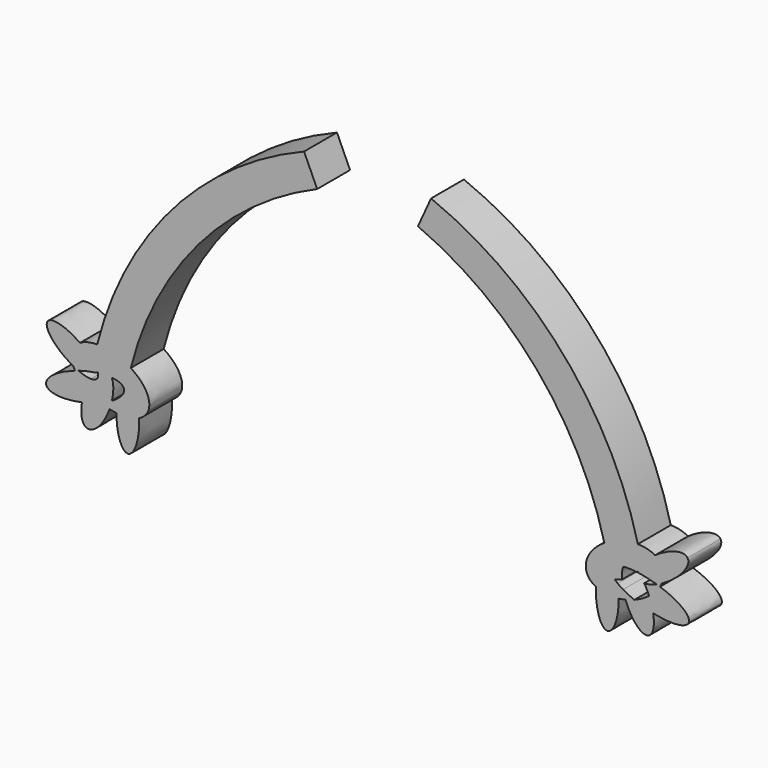
from build123d import *

# Parameters (mm, degrees)
F1_DEPTH = 5.588


with BuildPart() as f1:
    # F0 (on Front) → F1 (new body)
    with BuildSketch(Plane.XZ):
        with BuildLine():
            Line((32.2706997395, 11.8237007409), (36.8935018778, 12.8905009478))
            ThreePointArc((36.8935018778, 12.8905009478), (36.8110087462, 13.2342292177), (36.7259397745, 13.5773290723))
            add(Edge.make_bspline(
                [(36.7259397745, 13.5773290723), (34.3340010738, 13.6080468465), (32.1682575581, 12.2374034623)],
                knots=[4.1398736957, 4.1398736957, 4.1398736957, 5.0351295074, 5.0351295074, 5.0351295074], degree=2, weights=[1, 0.9014763473, 1]))
            ThreePointArc((32.1682575581, 12.2374034623), (32.2199801898, 12.0306762946), (32.2706997395, 11.8237007409))
        make_face()
        with BuildLine():
            ThreePointArc((36.7259397745, 13.5773290723), (36.8110087462, 13.2342292177), (36.8935018778, 12.8905009478))
            Line((36.8935018778, 12.8905009478), (32.2706997395, 11.8237007409))
            ThreePointArc((32.2706997395, 11.8237007409), (32.2199801898, 12.0306762946), (32.1682575581, 12.2374034623))
            add(Edge.make_bspline(
                [(32.1682575581, 12.2374034623), (28.9205076549, 10.1819860565), (29.7814980149, 7.9121002927)],
                knots=[5.0351295074, 5.0351295074, 5.0351295074, 6.2831853072, 6.2831853072, 6.2831853072], degree=2, weights=[1, 0.8115315094, 1]))
            add(Edge.make_bspline(
                [(29.7814980149, 7.9121002927), (30.0935316875, 7.0894653085), (31.0231862525, 6.6210745378)],
                knots=[0, 0, 0, 0.5104960555, 0.5104960555, 0.5104960555], degree=2, weights=[1, 0.9676007021, 1]))
            add(Edge.make_bspline(
                [(31.0231862525, 6.6210745378), (32.2803370197, 5.9876803301), (34.1259638549, 6.2135645276)],
                knots=[0.5104960555, 0.5104960555, 0.5104960555, 1.1889418798, 1.1889418798, 1.1889418798], degree=2, weights=[1, 0.9430135296, 1]))
            add(Edge.make_bspline(
                [(34.1259638549, 6.2135645276), (34.1243304614, 7.1393539704), (33.986892498, 7.9823561587)],
                knots=[1.5757090143, 1.5757090143, 1.5757090143, 1.9969423736, 1.9969423736, 1.9969423736], degree=2, weights=[1, 0.9779021758, 1]))
            add(Edge.make_bspline(
                [(33.5814264788, 8.3342957348), (33.7569586016, 8.1594602494), (33.986892498, 7.9823561587)],
                knots=[3.6789423363, 3.6789423363, 3.6789423363, 3.8326748164, 3.8326748164, 3.8326748164], degree=2, weights=[1, 0.9970472448, 1]))
            ThreePointArc((33.5814264788, 8.3342957349), (33.7430587819, 8.3767272254), (33.9042244499, 8.4208980334))
            ThreePointArc((33.9042244499, 8.4208980334), (34.2272864678, 8.5151058653), (34.5482281316, 8.6163018704))
            add(Edge.make_bspline(
                [(34.7502826908, 10.2419972443), (34.4767828785, 9.6352454307), (34.5482281316, 8.6163018704)],
                knots=[3.5532795904, 3.5532795904, 3.5532795904, 4.1157635759, 4.1157635759, 4.1157635759], degree=2, weights=[1, 0.9607114655, 1]))
            add(Edge.make_bspline(
                [(36.6366435764, 10.182329208), (35.5729011314, 10.3132979273), (34.7502826908, 10.2419972443)],
                knots=[1.9968428936, 1.9968428936, 1.9968428936, 2.4151242253, 2.4151242253, 2.4151242253], degree=2, weights=[1, 0.9782096903, 1]))
            add(Edge.make_bspline(
                [(36.6736091343, 10.3151708305), (36.6517615378, 10.247208944), (36.6366435764, 10.182329208)],
                knots=[2.6853839142, 2.6853839142, 2.6853839142, 2.7479252243, 2.7479252243, 2.7479252243], degree=2, weights=[1, 0.9995111129, 1]))
            add(Edge.make_bspline(
                [(39.0587814304, 13.001263099), (37.0867427344, 11.6003162638), (36.6736091343, 10.3151708305)],
                knots=[1.6170702637, 1.6170702637, 1.6170702637, 2.6853839142, 2.6853839142, 2.6853839142], degree=2, weights=[1, 0.8606982085, 1]))
            add(Edge.make_bspline(
                [(39.0587814304, 13.001263099), (38.1255784861, 13.559354621), (36.7259397745, 13.5773290723)],
                knots=[3.5920969612, 3.5920969612, 3.5920969612, 4.1398736957, 4.1398736957, 4.1398736957], degree=2, weights=[1, 0.9627264634, 1]))
        make_face()
        with BuildLine():
            add(Edge.make_bspline(
                [(36.7259397745, 13.5773290723), (34.3340010738, 13.6080468465), (32.1682575581, 12.2374034623)],
                knots=[4.1398736957, 4.1398736957, 4.1398736957, 5.0351295074, 5.0351295074, 5.0351295074], degree=2, weights=[1, 0.9014763473, 1]))
            ThreePointArc((36.7259397745, 13.5773290723), (26.5357798175, 33.0496078391), (8.6232991889, 45.7835011184))
            Line((8.6232991889, 45.7835011184), (6.8453005515, 41.8718978763))
            ThreePointArc((6.8453005515, 41.8718978763), (22.9723649253, 30.0160267189), (32.1682575581, 12.2374034623))
        make_face()
        with BuildLine():
            add(Edge.make_bspline(
                [(43.4721000493, 14.1350999475), (42.5506163385, 15.4818812905), (39.0587814304, 13.001263099)],
                knots=[0, 0, 0, 1.6170702637, 1.6170702637, 1.6170702637], degree=2, weights=[1, 0.690558678, 1]))
            add(Edge.make_bspline(
                [(39.9796777774, 9.9352008957), (40.8468053822, 11.9319554905), (39.0587814304, 13.001263099)],
                knots=[2.604464445, 2.604464445, 2.604464445, 3.5920969612, 3.5920969612, 3.5920969612], degree=2, weights=[1, 0.8805304081, 1]))
            add(Edge.make_bspline(
                [(39.9796777774, 9.9352008957), (44.6497104326, 12.413980328), (43.4721000493, 14.1350999475)],
                knots=[4.4248856689, 4.4248856689, 4.4248856689, 6.2831853072, 6.2831853072, 6.2831853072], degree=2, weights=[1, 0.5985152881, 1]))
        make_face()
        with BuildLine():
            add(Edge.make_bspline(
                [(39.9796777774, 9.9352008957), (40.8468053822, 11.9319554905), (39.0587814304, 13.001263099)],
                knots=[2.604464445, 2.604464445, 2.604464445, 3.5920969612, 3.5920969612, 3.5920969612], degree=2, weights=[1, 0.8805304081, 1]))
            add(Edge.make_bspline(
                [(39.0587814304, 13.001263099), (37.0867427344, 11.6003162638), (36.6736091343, 10.3151708305)],
                knots=[1.6170702637, 1.6170702637, 1.6170702637, 2.6853839142, 2.6853839142, 2.6853839142], degree=2, weights=[1, 0.8606982085, 1]))
            add(Edge.make_bspline(
                [(36.838546125, 10.1558680731), (36.7561354159, 10.2402088688), (36.6736091343, 10.3151708305)],
                knots=[2.3750268658, 2.3750268658, 2.3750268658, 2.4506633861, 2.4506633861, 2.4506633861], degree=2, weights=[1, 0.9992849748, 1]))
            add(Edge.make_bspline(
                [(37.6420765384, 10.020492761), (37.2334774045, 10.1010140748), (36.838546125, 10.1558680731)],
                knots=[1.8015665825, 1.8015665825, 1.8015665825, 1.9568242788, 1.9568242788, 1.9568242788], degree=2, weights=[1, 0.9969883938, 1]))
            add(Edge.make_bspline(
                [(39.2873464103, 9.604313109), (38.467052792, 9.8579173509), (37.6420765384, 10.020492761)],
                knots=[1.4900094279, 1.4900094279, 1.4900094279, 1.8015665825, 1.8015665825, 1.8015665825], degree=2, weights=[1, 0.9878910345, 1]))
            add(Edge.make_bspline(
                [(39.2873464103, 9.604313109), (39.6288573586, 9.748990969), (39.9796777774, 9.9352008957)],
                knots=[4.2244590735, 4.2244590735, 4.2244590735, 4.4248856689, 4.4248856689, 4.4248856689], degree=2, weights=[1, 0.9949828484, 1]))
        make_face()
        with BuildLine():
            add(Edge.make_bspline(
                [(39.7319677558, 9.459773657), (39.8761405135, 9.6967832669), (39.9796777774, 9.9352008957)],
                knots=[2.4760921827, 2.4760921827, 2.4760921827, 2.604464445, 2.604464445, 2.604464445], degree=2, weights=[1, 0.9979407774, 1]))
            add(Edge.make_bspline(
                [(39.2873464103, 9.604313109), (39.6288573586, 9.748990969), (39.9796777774, 9.9352008957)],
                knots=[4.2244590735, 4.2244590735, 4.2244590735, 4.4248856689, 4.4248856689, 4.4248856689], degree=2, weights=[1, 0.9949828484, 1]))
            add(Edge.make_bspline(
                [(39.7319677558, 9.459773657), (39.5117613547, 9.5349323646), (39.2873464103, 9.604313109)],
                knots=[1.4041305877, 1.4041305877, 1.4041305877, 1.4900094279, 1.4900094279, 1.4900094279], degree=2, weights=[1, 0.9990782447, 1]))
        make_face()
        with BuildLine():
            add(Edge.make_bspline(
                [(38.8016372647, 5.9750217773), (43.2541867053, 5.0072999504), (43.6518237169, 6.4967344439), (44.0494607285, 7.9861689374), (39.7319677558, 9.459773657)],
                knots=[4.8870250081, 4.8870250081, 4.8870250081, 6.2871704515, 6.2871704515, 7.6873158949, 7.6873158949, 7.6873158949], degree=2, weights=[1, 0.7647953367, 1, 0.7647953367, 1]))
            add(Edge.make_bspline(
                [(38.2513832681, 7.8754265107), (39.210650648, 8.6027659512), (39.7319677558, 9.459773657)],
                knots=[2.019377813, 2.019377813, 2.019377813, 2.4760921827, 2.4760921827, 2.4760921827], degree=2, weights=[1, 0.9740396059, 1]))
            add(Edge.make_bspline(
                [(38.8016372647, 5.9750217773), (38.6410074231, 6.9230354431), (38.2513832681, 7.8754265107)],
                knots=[1.1577399392, 1.1577399392, 1.1577399392, 1.650437424, 1.650437424, 1.650437424], degree=2, weights=[1, 0.9698092967, 1]))
        make_face()
        with BuildLine():
            add(Edge.make_bspline(
                [(38.2513832681, 7.8754265107), (39.210650648, 8.6027659512), (39.7319677558, 9.459773657)],
                knots=[2.019377813, 2.019377813, 2.019377813, 2.4760921827, 2.4760921827, 2.4760921827], degree=2, weights=[1, 0.9740396059, 1]))
            add(Edge.make_bspline(
                [(39.7319677558, 9.459773657), (39.5117613547, 9.5349323646), (39.2873464103, 9.604313109)],
                knots=[1.4041305877, 1.4041305877, 1.4041305877, 1.4900094279, 1.4900094279, 1.4900094279], degree=2, weights=[1, 0.9990782447, 1]))
            add(Edge.make_bspline(
                [(37.5898259242, 9.1787969257), (38.2981843104, 9.1852640083), (39.2873464103, 9.604313109)],
                knots=[3.6576642826, 3.6576642826, 3.6576642826, 4.2244590735, 4.2244590735, 4.2244590735], degree=2, weights=[1, 0.9601110043, 1]))
            add(Edge.make_bspline(
                [(38.2513832681, 7.8754265107), (37.9624894998, 8.5815938285), (37.5898259242, 9.1787969257)],
                knots=[1.650437424, 1.650437424, 1.650437424, 2.0190978507, 2.0190978507, 2.0190978507], degree=2, weights=[1, 0.9830592351, 1]))
        make_face()
        with BuildLine():
            add(Edge.make_bspline(
                [(31.0231862525, 6.6210745378), (32.2803370197, 5.9876803301), (34.1259638549, 6.2135645276)],
                knots=[0.5104960555, 0.5104960555, 0.5104960555, 1.1889418798, 1.1889418798, 1.1889418798], degree=2, weights=[1, 0.9430135296, 1]))
            add(Edge.make_bspline(
                [(31.0231862525, 6.6210745378), (30.8609649248, 2.0815590872), (32.4974887078, 1.866622695), (34.1340124909, 1.6516863028), (34.1259638549, 6.2135645276)],
                knots=[4.613210998, 4.613210998, 4.613210998, 6.2360526598, 6.2360526598, 7.8588943215, 7.8588943215, 7.8588943215], degree=2, weights=[1, 0.6884686478, 1, 0.6884686478, 1]))
        make_face()
        with BuildLine():
            add(Edge.make_bspline(
                [(38.8016372647, 5.9750217773), (38.6410074231, 6.9230354431), (38.2513832681, 7.8754265107)],
                knots=[1.1577399392, 1.1577399392, 1.1577399392, 1.650437424, 1.650437424, 1.650437424], degree=2, weights=[1, 0.9698092967, 1]))
            add(Edge.make_bspline(
                [(36.2437126455, 6.7579420356), (37.3562007183, 7.196677719), (38.2513832681, 7.8754265107)],
                knots=[1.5922240618, 1.5922240618, 1.5922240618, 2.019377813, 2.019377813, 2.019377813], degree=2, weights=[1, 0.9772790247, 1]))
            add(Edge.make_bspline(
                [(36.2437126455, 6.7579420356), (37.4688080387, 6.2647002976), (38.8016372647, 5.9750217773)],
                knots=[4.3929880742, 4.3929880742, 4.3929880742, 4.8870250081, 4.8870250081, 4.8870250081], degree=2, weights=[1, 0.9696457571, 1]))
        make_face()
        with BuildLine():
            add(Edge.make_bspline(
                [(35.0496863908, 6.3809924019), (36.1985024094, 3.2377777269), (37.7606059218, 3.068754155), (39.3227094342, 2.899730583), (38.8016372647, 5.9750217773)],
                knots=[4.703944968, 4.703944968, 4.703944968, 6.0724351072, 6.0724351072, 7.4409252464, 7.4409252464, 7.4409252464], degree=2, weights=[1, 0.7748964505, 1, 0.7748964505, 1]))
            add(Edge.make_bspline(
                [(36.2437126455, 6.7579420356), (37.4688080387, 6.2647002976), (38.8016372647, 5.9750217773)],
                knots=[4.3929880742, 4.3929880742, 4.3929880742, 4.8870250081, 4.8870250081, 4.8870250081], degree=2, weights=[1, 0.9696457571, 1]))
            add(Edge.make_bspline(
                [(35.0496863908, 6.3809924019), (35.6560069837, 6.5261665663), (36.2437126455, 6.7579420356)],
                knots=[1.3640671148, 1.3640671148, 1.3640671148, 1.5922240618, 1.5922240618, 1.5922240618], degree=2, weights=[1, 0.9935001046, 1]))
        make_face()
        with BuildLine():
            add(Edge.make_bspline(
                [(34.1259638549, 6.2135645276), (34.1243304614, 7.1393539704), (33.986892498, 7.9823561587)],
                knots=[1.5757090143, 1.5757090143, 1.5757090143, 1.9969423736, 1.9969423736, 1.9969423736], degree=2, weights=[1, 0.9779021758, 1]))
            add(Edge.make_bspline(
                [(34.1259638549, 6.2135645276), (34.58512877, 6.2697612063), (35.0496863908, 6.3809924019)],
                knots=[1.1889418798, 1.1889418798, 1.1889418798, 1.3640671148, 1.3640671148, 1.3640671148], degree=2, weights=[1, 0.9961688428, 1]))
            add(Edge.make_bspline(
                [(34.7193628832, 7.4945536546), (34.8463562994, 6.9373130979), (35.0496863908, 6.3809924019)],
                knots=[4.4171809306, 4.4171809306, 4.4171809306, 4.703944968, 4.703944968, 4.703944968], degree=2, weights=[1, 0.9897383966, 1]))
            add(Edge.make_bspline(
                [(33.986892498, 7.9823561587), (34.3069609657, 7.7358268919), (34.7193628832, 7.4945536546)],
                knots=[3.8326748164, 3.8326748164, 3.8326748164, 4.0462773342, 4.0462773342, 4.0462773342], degree=2, weights=[1, 0.9943021647, 1]))
        make_face()
        with BuildLine():
            add(Edge.make_bspline(
                [(35.0496863908, 6.3809924019), (35.6560069837, 6.5261665663), (36.2437126455, 6.7579420356)],
                knots=[1.3640671148, 1.3640671148, 1.3640671148, 1.5922240618, 1.5922240618, 1.5922240618], degree=2, weights=[1, 0.9935001046, 1]))
            add(Edge.make_bspline(
                [(34.7193628832, 7.4945536546), (35.3929708023, 7.1004634325), (36.2437126455, 6.7579420356)],
                knots=[4.0462773342, 4.0462773342, 4.0462773342, 4.3929880742, 4.3929880742, 4.3929880742], degree=2, weights=[1, 0.9850115505, 1]))
            add(Edge.make_bspline(
                [(34.7193628832, 7.4945536546), (34.8463562994, 6.9373130979), (35.0496863908, 6.3809924019)],
                knots=[4.4171809306, 4.4171809306, 4.4171809306, 4.703944968, 4.703944968, 4.703944968], degree=2, weights=[1, 0.9897383966, 1]))
        make_face()
    extrude(amount=F1_DEPTH)


with BuildPart() as f1b:
    # F0 (on Front) → F1, piece 2 (new body)
    with BuildSketch(Plane.XZ):
        with BuildLine():
            Line((-32.2706997395, 11.8237007409), (-36.8935018778, 12.8905009478))
            ThreePointArc((-36.8935018778, 12.8905009478), (-36.8110087462, 13.2342292177), (-36.7259397745, 13.5773290723))
            add(Edge.make_bspline(
                [(-36.7259397745, 13.5773290723), (-38.1255784861, 13.559354621), (-39.0587814304, 13.001263099)],
                knots=[2.1433116115, 2.1433116115, 2.1433116115, 2.691088346, 2.691088346, 2.691088346], degree=2, weights=[1, 0.9627264634, 1]))
            add(Edge.make_bspline(
                [(-36.6736091343, 10.3151708305), (-37.0867427344, 11.6003162638), (-39.0587814304, 13.001263099)],
                knots=[3.5978013929, 3.5978013929, 3.5978013929, 4.6661150434, 4.6661150434, 4.6661150434], degree=2, weights=[1, 0.8606982085, 1]))
            add(Edge.make_bspline(
                [(-36.6366435764, 10.182329208), (-36.6517615378, 10.247208944), (-36.6736091343, 10.3151708305)],
                knots=[3.5352600828, 3.5352600828, 3.5352600828, 3.5978013929, 3.5978013929, 3.5978013929], degree=2, weights=[1, 0.9995111129, 1]))
            add(Edge.make_bspline(
                [(-37.5898259242, 9.1787969257), (-36.4002747552, 9.167936709), (-36.6366435764, 10.182329208)],
                knots=[2.6255210246, 2.6255210246, 2.6255210246, 3.5352600828, 3.5352600828, 3.5352600828], degree=2, weights=[1, 0.8983183576, 1]))
            add(Edge.make_bspline(
                [(-37.5898259242, 9.1787969257), (-37.9624894998, 8.5815938285), (-38.2513832681, 7.8754265107)],
                knots=[4.2640874565, 4.2640874565, 4.2640874565, 4.6327478832, 4.6327478832, 4.6327478832], degree=2, weights=[1, 0.9830592351, 1]))
            add(Edge.make_bspline(
                [(-38.2513832681, 7.8754265107), (-37.3562007183, 7.196677719), (-36.2437126455, 6.7579420356)],
                knots=[4.2638074942, 4.2638074942, 4.2638074942, 4.6909612454, 4.6909612454, 4.6909612454], degree=2, weights=[1, 0.9772790247, 1]))
            add(Edge.make_bspline(
                [(-36.2437126455, 6.7579420356), (-35.3929708023, 7.1004634325), (-34.7193628832, 7.4945536546)],
                knots=[1.8901972329, 1.8901972329, 1.8901972329, 2.2369079729, 2.2369079729, 2.2369079729], degree=2, weights=[1, 0.9850115505, 1]))
            add(Edge.make_bspline(
                [(-34.7193628832, 7.4945536546), (-34.3138711823, 9.2738303121), (-34.7502826908, 10.2419972443)],
                knots=[1.8660043766, 1.8660043766, 1.8660043766, 2.7299057168, 2.7299057168, 2.7299057168], degree=2, weights=[1, 0.9081508434, 1]))
            add(Edge.make_bspline(
                [(-33.986892498, 7.9823561587), (-31.4271573207, 9.9539644252), (-34.7502826908, 10.2419972443)],
                knots=[2.4505104908, 2.4505104908, 2.4505104908, 3.8680610818, 3.8680610818, 3.8680610818], degree=2, weights=[1, 0.7591596108, 1]))
            add(Edge.make_bspline(
                [(-33.986892498, 7.9823561587), (-34.1243304614, 7.1393539704), (-34.1259638549, 6.2135645276)],
                knots=[4.2862429336, 4.2862429336, 4.2862429336, 4.7074762928, 4.7074762928, 4.7074762928], degree=2, weights=[1, 0.9779021758, 1]))
            add(Edge.make_bspline(
                [(-34.1259638549, 6.2135645276), (-32.2803370197, 5.9876803301), (-31.0231862525, 6.6210745378)],
                knots=[5.0942434274, 5.0942434274, 5.0942434274, 5.7726892517, 5.7726892517, 5.7726892517], degree=2, weights=[1, 0.9430135296, 1]))
            add(Edge.make_bspline(
                [(-31.0231862525, 6.6210745378), (-30.0935316875, 7.0894653085), (-29.7814980149, 7.9121002927)],
                knots=[5.7726892517, 5.7726892517, 5.7726892517, 6.2831853072, 6.2831853072, 6.2831853072], degree=2, weights=[1, 0.9676007021, 1]))
            add(Edge.make_bspline(
                [(-29.7814980149, 7.9121002927), (-28.9205076549, 10.1819860565), (-32.1682575581, 12.2374034623)],
                knots=[0, 0, 0, 1.2480557998, 1.2480557998, 1.2480557998], degree=2, weights=[1, 0.8115315094, 1]))
            ThreePointArc((-32.1682575581, 12.2374034623), (-32.2199801898, 12.0306762946), (-32.2706997395, 11.8237007409))
        make_face()
        with BuildLine():
            ThreePointArc((-36.7259397745, 13.5773290723), (-36.8110087462, 13.2342292177), (-36.8935018778, 12.8905009478))
            Line((-36.8935018778, 12.8905009478), (-32.2706997395, 11.8237007409))
            ThreePointArc((-32.2706997395, 11.8237007409), (-32.2199801898, 12.0306762946), (-32.1682575581, 12.2374034623))
            add(Edge.make_bspline(
                [(-32.1682575581, 12.2374034623), (-34.3340010738, 13.6080468465), (-36.7259397745, 13.5773290723)],
                knots=[1.2480557998, 1.2480557998, 1.2480557998, 2.1433116115, 2.1433116115, 2.1433116115], degree=2, weights=[1, 0.9014763473, 1]))
        make_face()
        with BuildLine():
            ThreePointArc((-8.6232991889, 45.7835011184), (-26.5357798175, 33.0496078391), (-36.7259397745, 13.5773290723))
            add(Edge.make_bspline(
                [(-32.1682575581, 12.2374034623), (-34.3340010738, 13.6080468465), (-36.7259397745, 13.5773290723)],
                knots=[1.2480557998, 1.2480557998, 1.2480557998, 2.1433116115, 2.1433116115, 2.1433116115], degree=2, weights=[1, 0.9014763473, 1]))
            ThreePointArc((-32.1682575581, 12.2374034623), (-22.9723649253, 30.0160267189), (-6.8453005515, 41.8718978763))
            Line((-6.8453005515, 41.8718978763), (-8.6232991889, 45.7835011184))
        make_face()
        with BuildLine():
            add(Edge.make_bspline(
                [(-36.6736091343, 10.3151708305), (-37.0867427344, 11.6003162638), (-39.0587814304, 13.001263099)],
                knots=[3.5978013929, 3.5978013929, 3.5978013929, 4.6661150434, 4.6661150434, 4.6661150434], degree=2, weights=[1, 0.8606982085, 1]))
            add(Edge.make_bspline(
                [(-39.0587814304, 13.001263099), (-39.8198979479, 12.5460859285), (-40.0939062238, 11.8236998096)],
                knots=[2.691088346, 2.691088346, 2.691088346, 3.1415926536, 3.1415926536, 3.1415926536], degree=2, weights=[1, 0.974737819, 1]))
            add(Edge.make_bspline(
                [(-40.0939062238, 11.8236998096), (-40.4230078995, 10.9560673212), (-39.9796777774, 9.9352008957)],
                knots=[3.1415926536, 3.1415926536, 3.1415926536, 3.6787208622, 3.6787208622, 3.6787208622], degree=2, weights=[1, 0.9641529012, 1]))
            add(Edge.make_bspline(
                [(-39.9796777774, 9.9352008957), (-39.6288573586, 9.748990969), (-39.2873464103, 9.604313109)],
                knots=[1.8582996383, 1.8582996383, 1.8582996383, 2.0587262337, 2.0587262337, 2.0587262337], degree=2, weights=[1, 0.9949828484, 1]))
            add(Edge.make_bspline(
                [(-36.838546125, 10.1558680731), (-38.045603473, 9.9882137871), (-39.2873464103, 9.604313109)],
                knots=[4.3263610283, 4.3263610283, 4.3263610283, 4.7931758793, 4.7931758793, 4.7931758793], degree=2, weights=[1, 0.9728839277, 1]))
            add(Edge.make_bspline(
                [(-36.6736091343, 10.3151708305), (-36.7561354159, 10.2402088688), (-36.838546125, 10.1558680731)],
                knots=[3.8325219211, 3.8325219211, 3.8325219211, 3.9081584414, 3.9081584414, 3.9081584414], degree=2, weights=[1, 0.9992849748, 1]))
        make_face()
        with BuildLine():
            add(Edge.make_bspline(
                [(-39.0587814304, 13.001263099), (-39.8198979479, 12.5460859285), (-40.0939062238, 11.8236998096)],
                knots=[2.691088346, 2.691088346, 2.691088346, 3.1415926536, 3.1415926536, 3.1415926536], degree=2, weights=[1, 0.974737819, 1]))
            add(Edge.make_bspline(
                [(-39.0587814304, 13.001263099), (-42.5506163385, 15.4818812905), (-43.4721000493, 14.1350999475)],
                knots=[4.6661150434, 4.6661150434, 4.6661150434, 6.2831853072, 6.2831853072, 6.2831853072], degree=2, weights=[1, 0.690558678, 1]))
            add(Edge.make_bspline(
                [(-43.4721000493, 14.1350999475), (-44.6497104326, 12.413980328), (-39.9796777774, 9.9352008957)],
                knots=[0, 0, 0, 1.8582996383, 1.8582996383, 1.8582996383], degree=2, weights=[1, 0.5985152881, 1]))
            add(Edge.make_bspline(
                [(-40.0939062238, 11.8236998096), (-40.4230078995, 10.9560673212), (-39.9796777774, 9.9352008957)],
                knots=[3.1415926536, 3.1415926536, 3.1415926536, 3.6787208622, 3.6787208622, 3.6787208622], degree=2, weights=[1, 0.9641529012, 1]))
        make_face()
        with BuildLine():
            add(Edge.make_bspline(
                [(-34.1259638549, 6.2135645276), (-34.1340124909, 1.6516863028), (-32.4974887078, 1.866622695), (-30.8609649248, 2.0815590872), (-31.0231862525, 6.6210745378)],
                knots=[4.7074762928, 4.7074762928, 4.7074762928, 6.3303179546, 6.3303179546, 7.9531596163, 7.9531596163, 7.9531596163], degree=2, weights=[1, 0.6884686478, 1, 0.6884686478, 1]))
            add(Edge.make_bspline(
                [(-34.1259638549, 6.2135645276), (-32.2803370197, 5.9876803301), (-31.0231862525, 6.6210745378)],
                knots=[5.0942434274, 5.0942434274, 5.0942434274, 5.7726892517, 5.7726892517, 5.7726892517], degree=2, weights=[1, 0.9430135296, 1]))
        make_face()
        with BuildLine():
            add(Edge.make_bspline(
                [(-39.9796777774, 9.9352008957), (-39.6288573586, 9.748990969), (-39.2873464103, 9.604313109)],
                knots=[1.8582996383, 1.8582996383, 1.8582996383, 2.0587262337, 2.0587262337, 2.0587262337], degree=2, weights=[1, 0.9949828484, 1]))
            add(Edge.make_bspline(
                [(-39.9796777774, 9.9352008957), (-39.8761405135, 9.6967832669), (-39.7319677558, 9.459773657)],
                knots=[3.6787208622, 3.6787208622, 3.6787208622, 3.8070931244, 3.8070931244, 3.8070931244], degree=2, weights=[1, 0.9979407774, 1]))
            add(Edge.make_bspline(
                [(-39.2873464103, 9.604313109), (-39.5117613547, 9.5349323646), (-39.7319677558, 9.459773657)],
                knots=[4.7931758793, 4.7931758793, 4.7931758793, 4.8790547195, 4.8790547195, 4.8790547195], degree=2, weights=[1, 0.9990782447, 1]))
        make_face()
        with BuildLine():
            add(Edge.make_bspline(
                [(-35.0496863908, 6.3809924019), (-34.58512877, 6.2697612063), (-34.1259638549, 6.2135645276)],
                knots=[4.9191181924, 4.9191181924, 4.9191181924, 5.0942434274, 5.0942434274, 5.0942434274], degree=2, weights=[1, 0.9961688428, 1]))
            add(Edge.make_bspline(
                [(-33.986892498, 7.9823561587), (-34.1243304614, 7.1393539704), (-34.1259638549, 6.2135645276)],
                knots=[4.2862429336, 4.2862429336, 4.2862429336, 4.7074762928, 4.7074762928, 4.7074762928], degree=2, weights=[1, 0.9779021758, 1]))
            add(Edge.make_bspline(
                [(-34.7193628832, 7.4945536546), (-34.3069609657, 7.7358268919), (-33.986892498, 7.9823561587)],
                knots=[2.2369079729, 2.2369079729, 2.2369079729, 2.4505104908, 2.4505104908, 2.4505104908], degree=2, weights=[1, 0.9943021647, 1]))
            add(Edge.make_bspline(
                [(-35.0496863908, 6.3809924019), (-34.8463562994, 6.9373130979), (-34.7193628832, 7.4945536546)],
                knots=[1.5792403392, 1.5792403392, 1.5792403392, 1.8660043766, 1.8660043766, 1.8660043766], degree=2, weights=[1, 0.9897383966, 1]))
        make_face()
        with BuildLine():
            add(Edge.make_bspline(
                [(-39.7319677558, 9.459773657), (-39.210650648, 8.6027659512), (-38.2513832681, 7.8754265107)],
                knots=[3.8070931244, 3.8070931244, 3.8070931244, 4.2638074942, 4.2638074942, 4.2638074942], degree=2, weights=[1, 0.9740396059, 1]))
            add(Edge.make_bspline(
                [(-39.7319677558, 9.459773657), (-44.0494607285, 7.9861689374), (-43.6518237169, 6.4967344439), (-43.2541867053, 5.0072999504), (-38.8016372647, 5.9750217773)],
                knots=[4.8790547195, 4.8790547195, 4.8790547195, 6.2792001629, 6.2792001629, 7.6793456062, 7.6793456062, 7.6793456062], degree=2, weights=[1, 0.7647953367, 1, 0.7647953367, 1]))
            add(Edge.make_bspline(
                [(-38.2513832681, 7.8754265107), (-38.6410074231, 6.9230354431), (-38.8016372647, 5.9750217773)],
                knots=[4.6327478832, 4.6327478832, 4.6327478832, 5.125445368, 5.125445368, 5.125445368], degree=2, weights=[1, 0.9698092967, 1]))
        make_face()
        with BuildLine():
            add(Edge.make_bspline(
                [(-39.2873464103, 9.604313109), (-39.5117613547, 9.5349323646), (-39.7319677558, 9.459773657)],
                knots=[4.7931758793, 4.7931758793, 4.7931758793, 4.8790547195, 4.8790547195, 4.8790547195], degree=2, weights=[1, 0.9990782447, 1]))
            add(Edge.make_bspline(
                [(-39.7319677558, 9.459773657), (-39.210650648, 8.6027659512), (-38.2513832681, 7.8754265107)],
                knots=[3.8070931244, 3.8070931244, 3.8070931244, 4.2638074942, 4.2638074942, 4.2638074942], degree=2, weights=[1, 0.9740396059, 1]))
            add(Edge.make_bspline(
                [(-37.5898259242, 9.1787969257), (-37.9624894998, 8.5815938285), (-38.2513832681, 7.8754265107)],
                knots=[4.2640874565, 4.2640874565, 4.2640874565, 4.6327478832, 4.6327478832, 4.6327478832], degree=2, weights=[1, 0.9830592351, 1]))
            add(Edge.make_bspline(
                [(-39.2873464103, 9.604313109), (-38.2981843104, 9.1852640083), (-37.5898259242, 9.1787969257)],
                knots=[2.0587262337, 2.0587262337, 2.0587262337, 2.6255210246, 2.6255210246, 2.6255210246], degree=2, weights=[1, 0.9601110043, 1]))
        make_face()
        with BuildLine():
            add(Edge.make_bspline(
                [(-38.8016372647, 5.9750217773), (-39.3227094342, 2.899730583), (-37.7606059218, 3.068754155), (-36.1985024094, 3.2377777269), (-35.0496863908, 6.3809924019)],
                knots=[5.125445368, 5.125445368, 5.125445368, 6.4939355072, 6.4939355072, 7.8624256464, 7.8624256464, 7.8624256464], degree=2, weights=[1, 0.7748964505, 1, 0.7748964505, 1]))
            add(Edge.make_bspline(
                [(-36.2437126455, 6.7579420356), (-35.6560069837, 6.5261665663), (-35.0496863908, 6.3809924019)],
                knots=[4.6909612454, 4.6909612454, 4.6909612454, 4.9191181924, 4.9191181924, 4.9191181924], degree=2, weights=[1, 0.9935001046, 1]))
            add(Edge.make_bspline(
                [(-38.8016372647, 5.9750217773), (-37.4688080387, 6.2647002976), (-36.2437126455, 6.7579420356)],
                knots=[1.3961602991, 1.3961602991, 1.3961602991, 1.8901972329, 1.8901972329, 1.8901972329], degree=2, weights=[1, 0.9696457571, 1]))
        make_face()
        with BuildLine():
            add(Edge.make_bspline(
                [(-36.2437126455, 6.7579420356), (-35.6560069837, 6.5261665663), (-35.0496863908, 6.3809924019)],
                knots=[4.6909612454, 4.6909612454, 4.6909612454, 4.9191181924, 4.9191181924, 4.9191181924], degree=2, weights=[1, 0.9935001046, 1]))
            add(Edge.make_bspline(
                [(-35.0496863908, 6.3809924019), (-34.8463562994, 6.9373130979), (-34.7193628832, 7.4945536546)],
                knots=[1.5792403392, 1.5792403392, 1.5792403392, 1.8660043766, 1.8660043766, 1.8660043766], degree=2, weights=[1, 0.9897383966, 1]))
            add(Edge.make_bspline(
                [(-36.2437126455, 6.7579420356), (-35.3929708023, 7.1004634325), (-34.7193628832, 7.4945536546)],
                knots=[1.8901972329, 1.8901972329, 1.8901972329, 2.2369079729, 2.2369079729, 2.2369079729], degree=2, weights=[1, 0.9850115505, 1]))
        make_face()
        with BuildLine():
            add(Edge.make_bspline(
                [(-38.2513832681, 7.8754265107), (-38.6410074231, 6.9230354431), (-38.8016372647, 5.9750217773)],
                knots=[4.6327478832, 4.6327478832, 4.6327478832, 5.125445368, 5.125445368, 5.125445368], degree=2, weights=[1, 0.9698092967, 1]))
            add(Edge.make_bspline(
                [(-38.8016372647, 5.9750217773), (-37.4688080387, 6.2647002976), (-36.2437126455, 6.7579420356)],
                knots=[1.3961602991, 1.3961602991, 1.3961602991, 1.8901972329, 1.8901972329, 1.8901972329], degree=2, weights=[1, 0.9696457571, 1]))
            add(Edge.make_bspline(
                [(-38.2513832681, 7.8754265107), (-37.3562007183, 7.196677719), (-36.2437126455, 6.7579420356)],
                knots=[4.2638074942, 4.2638074942, 4.2638074942, 4.6909612454, 4.6909612454, 4.6909612454], degree=2, weights=[1, 0.9772790247, 1]))
        make_face()
    extrude(amount=F1_DEPTH)


solid = Compound([f1.part, f1b.part])
